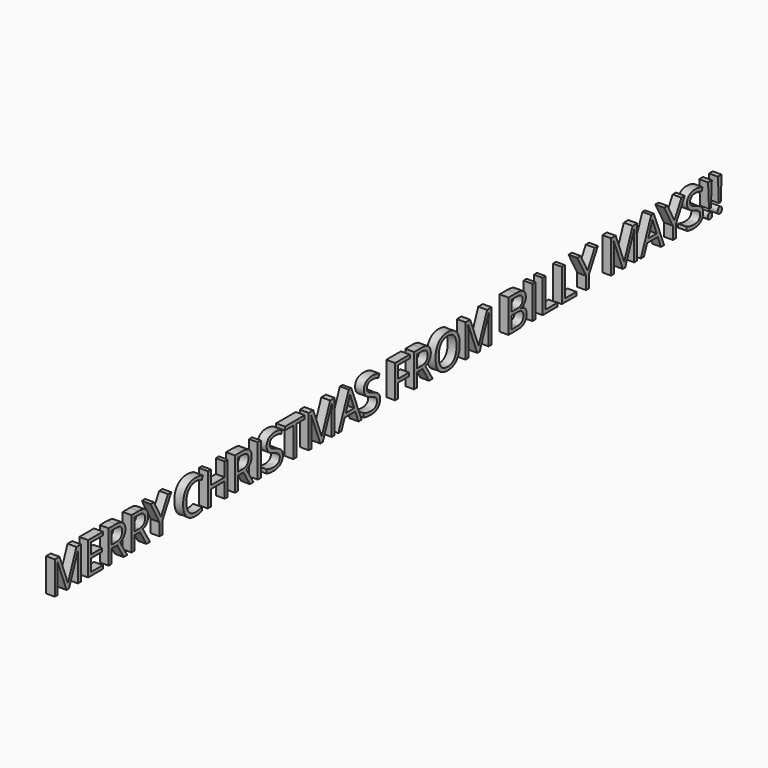
from build123d import *

# Parameters (mm, degrees)
F0_TEXT_SIZE = 132.6330678744
F1_DEPTH     = 25.4


# Not quite as in the source:
# - Text() gives the source's letters only with a copy of the font that has no kerning and outlines rounded to 1/6400 em; it was checked with that copy


with BuildPart() as f1:
    # F0 (on Right) → F1 (new body)
    with BuildSketch(Plane.YZ):
        with Locations((-662.7642810345, -68.6586368829)):
            Text('MERRY CHRISTMAS FROM BILLY MAYS!!', F0_TEXT_SIZE, font='Open Sans', text_align=(TextAlign.LEFT, TextAlign.BOTTOM))
    extrude(amount=F1_DEPTH)


solid = f1.part
